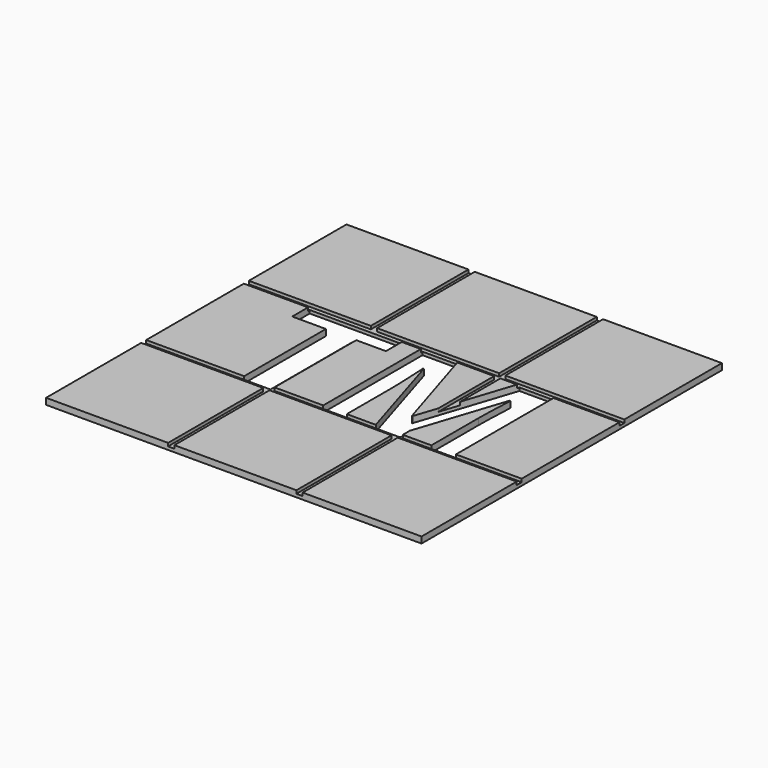
from build123d import *

# Parameters (mm, degrees)
F0_W         = 120
F0_H         = 120
F1_DEPTH     = 2
F2_TEXT_SIZE = 55.5555555556
F3_DEPTH     = 25
F4_W         = 49
F4_H         = 2
F4_W_2       = 2
F4_H_2       = 46.1985447407
F4_W_3       = 39
F4_H_3       = 39
F4_H_4       = 47.617426157
F4_W_4       = 44.1755156983
F4_W_5       = 48
F4_H_5       = 49.4188814163
F4_W_6       = 52.8244843017
F4_H_6       = 48
F5_DEPTH     = 1


# Not quite as in the source:
# - Text() gives the source's letters only with a copy of the font that has no kerning and outlines rounded to 1/6400 em; it was checked with that copy


with BuildPart() as f1:
    # F0 (on Top) → F1 (new body)
    with BuildSketch(Plane.XY):
        with Locations((-1, 0)):
            Rectangle(F0_W, F0_H)
    extrude(amount=F1_DEPTH)

    # F2 (on face) → F3 (cut)
    with BuildSketch(Plane.XY.offset(2)):
        with Locations((-41.57986, -20)):
            Text('TM', F2_TEXT_SIZE, font='Open Sans', font_style=FontStyle.BOLD, text_align=(TextAlign.LEFT, TextAlign.BOTTOM))
    extrude(amount=-F3_DEPTH, mode=Mode.SUBTRACT)

    # F4 (on face) → F5 (cut)
    with BuildSketch(Plane.XY.offset(2)):
        with Locations((-46.5, 20)):
            Rectangle(F4_W, F4_H)
        with Locations((-21, 44.0992723703)):
            Rectangle(F4_W_2, F4_H_2)
        with Locations((-21, 20)):
            Rectangle(F4_W_2, F4_H)
        with Locations((-0.5, 20)):
            Rectangle(F4_W_3, F4_H)
        with Locations((-21, -0.5)):
            Rectangle(F4_W_2, F4_H_3)
        with Locations((20, 44.8087130785)):
            Rectangle(F4_W_2, F4_H_4)
        with Locations((20, 20)):
            Rectangle(F4_W_2, F4_H)
        with Locations((-44.0877578491, -21)):
            Rectangle(F4_W_4, F4_H)
        with Locations((-21, -21)):
            Rectangle(F4_W_2, F4_H)
        with Locations((45, 20)):
            Rectangle(F4_W_5, F4_H)
        with Locations((20, -0.5)):
            Rectangle(F4_W_2, F4_H_3)
        with Locations((-0.5, -21)):
            Rectangle(F4_W_3, F4_H)
        with Locations((-21, -46.7094407082)):
            Rectangle(F4_W_2, F4_H_5)
        with Locations((20, -21)):
            Rectangle(F4_W_2, F4_H)
        with Locations((47.4122421509, -21)):
            Rectangle(F4_W_6, F4_H)
        with Locations((20, -46)):
            Rectangle(F4_W_2, F4_H_6)
    extrude(amount=-F5_DEPTH, mode=Mode.SUBTRACT)


solid = f1.part
